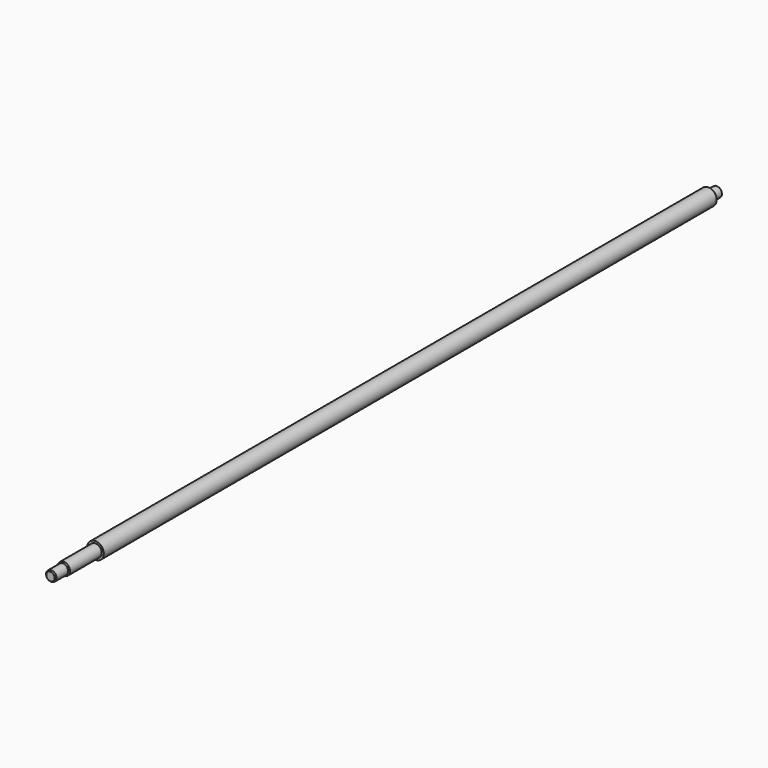
from build123d import *

# Parameters (mm, degrees)
F2_SIZE = 0.99999


# Not quite as in the source:
# - a fillet or chamfer is up to 0.001 mm smaller than in the source, because OpenCascade refuses the exact size


with BuildPart() as f1:
    # F0 (on Right) → F1 (revolve)
    with BuildSketch(Plane.YZ):
        Polygon((0, 5), (0, 0), (800, 0), (800, 5), (789, 5), (789, 8), (54, 8), (54, 6), (15, 6), (15, 5), align=None)
    revolve(axis=Axis((0, 344.1624132916, 0), (0, 1, 0)))

    # F2 (size 1 in the source; OpenCascade refuses exactly that, so slightly less here)
    f2_edges = [f1.edges().sort_by_distance(p)[0] for p in [
        (0, 0, -5),
        (0, 15, -6),
        (0, 800, -5),
    ]]
    chamfer(f2_edges, length=F2_SIZE)


solid = f1.part
